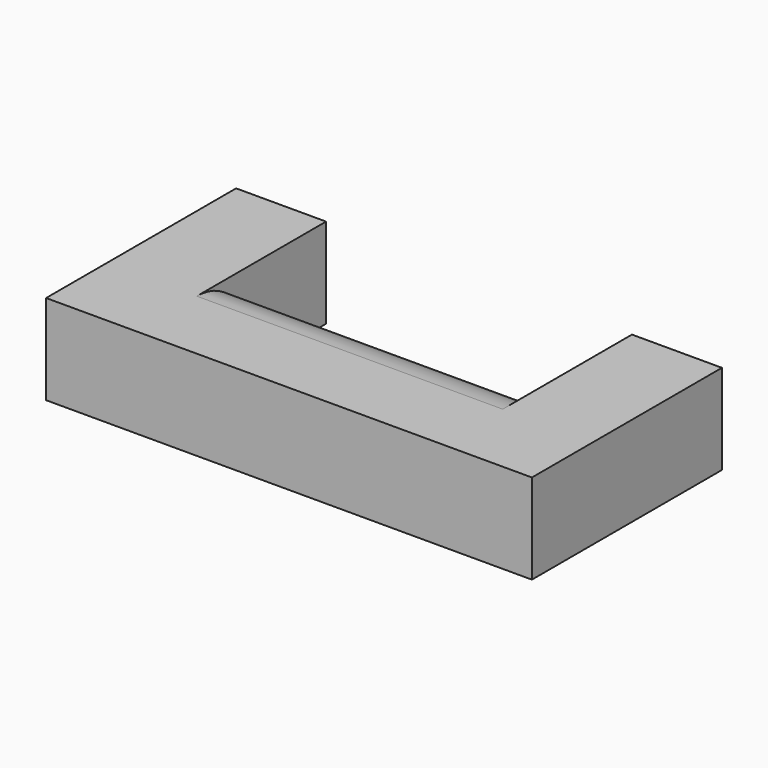
from build123d import *

# Parameters (mm, degrees)
F0_W        = 135
F0_H        = 25
F1_DEPTH    = 38
F2_W        = 25
F2_H        = 25
F3_DEPTH    = 28
F4_T1_DEPTH = 85


# Not quite as in the source:
# - a fillet or chamfer that OpenCascade refuses, or shapes differently, is made with other operations: its cross-section is extruded or revolved along the edge and cut away or added


with BuildPart() as f1:
    # F0 (on Front) → F1 (new body)
    with BuildSketch(Plane.XZ):
        with Locations((67.5, -12.5)):
            Rectangle(F0_W, F0_H)
    extrude(amount=F1_DEPTH)

    # F2 (on face) → F3 (join)
    with BuildSketch(Plane(origin=(0, 0, 0), x_dir=(-1, 0, 0), z_dir=(0, 1, 0))):
        with Locations((-122.5, -12.5)):
            Rectangle(F2_W, F2_H)
        with Locations((-12.5, -12.5)):
            Rectangle(F2_W, F2_H)
    extrude(amount=F3_DEPTH)

    # F4: fillet of radius 16.8994949366 on 2 edges, made by hand

    # F4_s2 → F4_t1 (cut)
    with BuildSketch(Plane.YZ.offset(25)):
        with BuildLine():
            ThreePointArc((-16.8994949366, 0), (-4.9497474683, -4.9497474683), (0, -16.8994949366))
            Line((0, -16.8994949366), (0, 0))
            Line((0, 0), (-16.8994949366, 0))
        make_face()
        with BuildLine():
            ThreePointArc((-16.8994949366, -25), (-4.9497474683, -20.0502525317), (0, -8.1005050634))
            Line((0, -8.1005050634), (0, -25))
            Line((0, -25), (-16.8994949366, -25))
        make_face()
    extrude(amount=F4_T1_DEPTH, mode=Mode.SUBTRACT)


solid = f1.part
